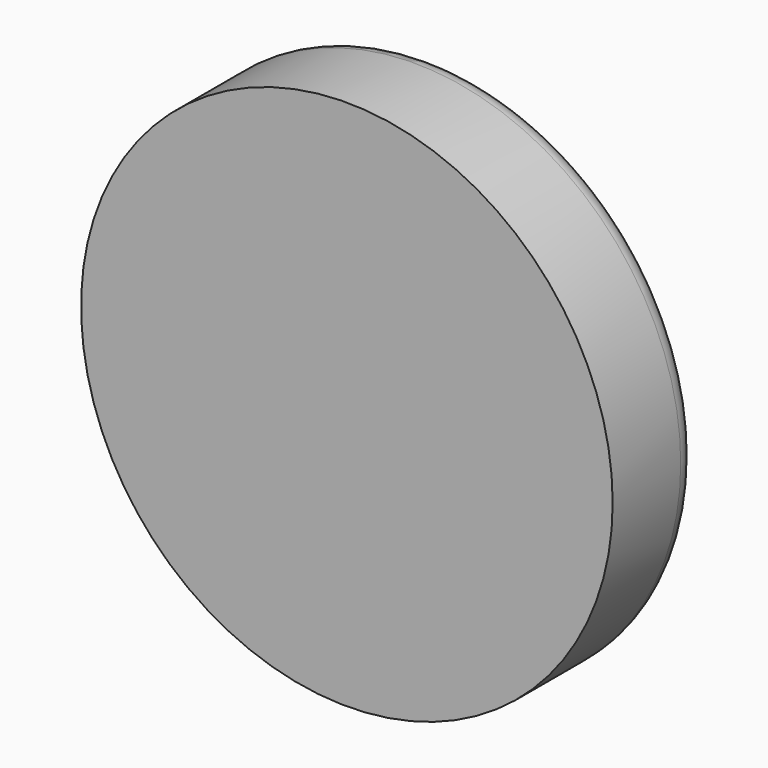
from build123d import *

# Parameters (mm, degrees)
F0_R     = 63.5
F1_DEPTH = 25.4
F4_R     = 5.08


# Not quite as in the source:
# - the program builds the solid bodies; features that only make, move or delete a surface that nothing else refers to are left out


with BuildPart() as f1:
    # F0 (on Front) → F1 (new body)
    with BuildSketch(Plane.XZ):
        Circle(F0_R)
    extrude(amount=F1_DEPTH)

    # F4
    f4_edges = [f1.edges().sort_by_distance(p)[0] for p in [
        (-63.5, 0, 0),
    ]]
    fillet(f4_edges, radius=F4_R)


solid = f1.part
